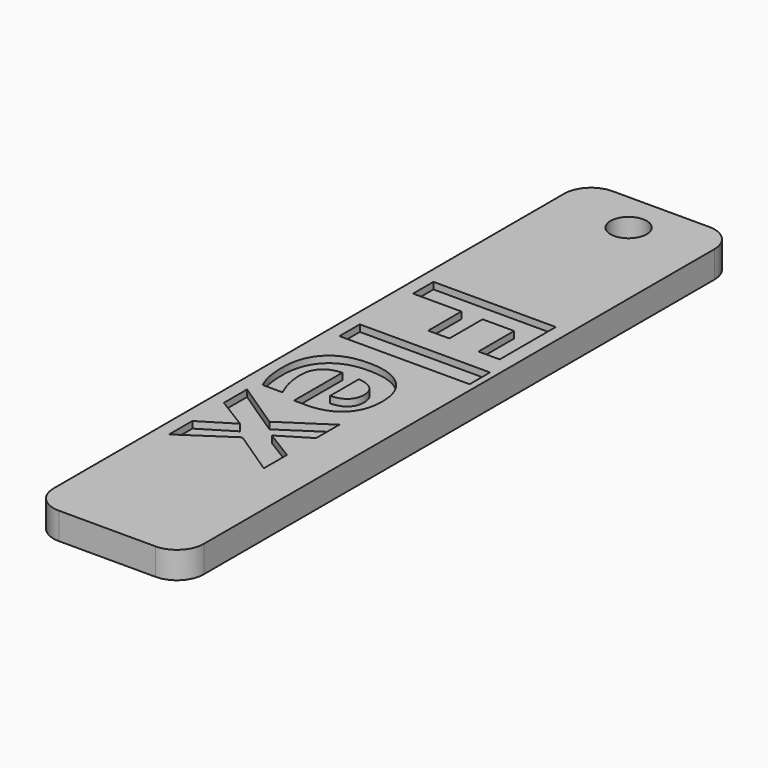
from build123d import *

# Parameters (mm, degrees)
F0_W         = 11.2
F0_H         = 51.6
F0_W_2       = 9.7091145833
F0_H_2       = 1.9026909722
F0_R         = 1.35
F0_TEXT_SIZE = 12.7777777778
F1_DEPTH     = 2
F2_DEPTH     = 0.5
F3_R         = 2


# Not quite as in the source:
# - a feature names something its author has since deleted; it is built from what else it names
# - Text() gives the source's letters only with a copy of the font that has no kerning and outlines rounded to 1/6400 em; it was checked with that copy


with BuildPart() as f1:
    # F0 (on Top) → F1 (new body)
    with BuildSketch(Plane.XY):
        with Locations((-43.6647401989, 53.6327249827)):
            Rectangle(F0_W, F0_H)
        Polygon((-48.2647401989, 46.6167961633), (-44.7029346433, 44.2509107466), (-41.2888721433, 46.4970044966), (-41.2888721433, 44.3387579688), (-43.51100756, 42.9851121355), (-41.2888721433, 41.6194871355), (-41.2888721433, 39.45924408), (-44.7029346433, 41.7312926911), (-48.2647401989, 39.3534281077), (-48.2647401989, 41.5196607466), (-45.8748964489, 42.9851121355), (-48.2647401989, 44.4565531077), align=None, mode=Mode.SUBTRACT)
        with BuildLine():
            add(Edge.make_bspline(
                [(-48.2687332544, 48.6871954688), (-48.3905214489, 49.2542093577), (-48.3905214489, 50.0727857466)],
                knots=[0, 0, 0, 1, 1, 1], degree=2))
            add(Edge.make_bspline(
                [(-48.3905214489, 50.0727857466), (-48.3905214489, 51.7558586633), (-47.4601395044, 52.7042093577)],
                knots=[0, 0, 0, 1, 1, 1], degree=2))
            add(Edge.make_bspline(
                [(-47.4601395044, 52.7042093577), (-46.52975756, 53.6525600522), (-44.8267193655, 53.6525600522)],
                knots=[0, 0, 0, 1, 1, 1], degree=2))
            add(Edge.make_bspline(
                [(-44.8267193655, 53.6525600522), (-43.0737679766, 53.6525600522), (-42.1164329072, 52.7760843577)],
                knots=[0, 0, 0, 1, 1, 1], degree=2))
            add(Edge.make_bspline(
                [(-42.1164329072, 52.7760843577), (-41.1590978377, 51.8996086633), (-41.1590978377, 50.3522996355)],
                knots=[0, 0, 0, 1, 1, 1], degree=2))
            add(Edge.make_bspline(
                [(-41.1590978377, 50.3522996355), (-41.1590978377, 48.87486908), (-42.0006342961, 48.0513013716)],
                knots=[0, 0, 0, 1, 1, 1], degree=2))
            add(Edge.make_bspline(
                [(-42.0006342961, 48.0513013716), (-42.8421707544, 47.2277336633), (-44.3275874211, 47.2277336633)],
                knots=[0, 0, 0, 1, 1, 1], degree=2))
            Line((-44.3275874211, 47.2277336633), (-45.2519797822, 47.2277336633))
            Line((-45.2519797822, 47.2277336633), (-45.2519797822, 51.7259107466))
            add(Edge.make_bspline(
                [(-45.2519797822, 51.7259107466), (-46.06257006, 51.6939663022), (-46.5177783933, 51.2447475522)],
                knots=[0, 0, 0, 1, 1, 1], degree=2))
            add(Edge.make_bspline(
                [(-46.5177783933, 51.2447475522), (-46.9729867266, 50.7955288022), (-46.9729867266, 49.9849385244)],
                knots=[0, 0, 0, 1, 1, 1], degree=2))
            add(Edge.make_bspline(
                [(-46.9729867266, 49.9849385244), (-46.9729867266, 49.3540357466), (-46.8422141572, 48.7930114411)],
                knots=[0, 0, 0, 1, 1, 1], degree=2))
            add(Edge.make_bspline(
                [(-46.8422141572, 48.7930114411), (-46.7114415877, 48.2319871355), (-46.4239415877, 47.6210496355)],
                knots=[0, 0, 0, 1, 1, 1], degree=2))
            Line((-46.4239415877, 47.6210496355), (-47.8973790877, 47.6210496355))
            add(Edge.make_bspline(
                [(-47.8973790877, 47.6210496355), (-48.14694506, 48.12018158), (-48.2687332544, 48.6871954688)],
                knots=[0, 0, 0, 1, 1, 1], degree=2))
        make_face(mode=Mode.SUBTRACT)
        Polygon((-44.6590110322, 62.0898864411), (-48.2647401989, 62.0898864411), (-48.2647401989, 63.9925774133), (-39.1426047822, 63.9925774133), (-39.1426047822, 58.7636711633), (-40.7278478377, 58.7636711633), (-40.7278478377, 62.0898864411), (-43.07975756, 62.0898864411), (-43.07975756, 58.9952683855), (-44.6590110322, 58.9952683855), align=None, mode=Mode.SUBTRACT)
        with Locations((-43.4101829072, 56.1771694272)):
            Rectangle(F0_W_2, F0_H_2, mode=Mode.SUBTRACT)
        with Locations((-43.6647401989, 76.4327249827)):
            Circle(F0_R, mode=Mode.SUBTRACT)
        with Locations(Location((-48.2647401989, 65.1405808855), (0, 0, -90))):
            Text('Flex', F0_TEXT_SIZE, font='Open Sans', font_style=FontStyle.BOLD, text_align=(TextAlign.LEFT, TextAlign.BOTTOM))
        with BuildLine():
            add(Edge.make_bspline(
                [(-42.8960770044, 49.3799906077), (-42.5127436711, 49.7353725522), (-42.5127436711, 50.3403204688)],
                knots=[0, 0, 0, 1, 1, 1], degree=2))
            add(Edge.make_bspline(
                [(-42.5127436711, 50.3403204688), (-42.5127436711, 50.9452683855), (-42.8960770044, 51.2886711633)],
                knots=[0, 0, 0, 1, 1, 1], degree=2))
            add(Edge.make_bspline(
                [(-42.8960770044, 51.2886711633), (-43.2794103377, 51.6320739411), (-43.9841846433, 51.6819871355)],
                knots=[0, 0, 0, 1, 1, 1], degree=2))
            Line((-43.9841846433, 51.6819871355), (-43.9841846433, 49.0106329688))
            add(Edge.make_bspline(
                [(-43.9841846433, 49.0106329688), (-43.2794103377, 49.0246086633), (-42.8960770044, 49.3799906077)],
                knots=[0, 0, 0, 1, 1, 1], degree=2))
        make_face()
    extrude(amount=-F1_DEPTH)

    # F0 (on Top) → F2 (cut)
    with BuildSketch(Plane.XY):
        with Locations(Location((-48.2647401989, 65.1405808855), (0, 0, -90))):
            Text('Flex', F0_TEXT_SIZE, font='Open Sans', font_style=FontStyle.BOLD, text_align=(TextAlign.LEFT, TextAlign.BOTTOM))
    extrude(amount=-F2_DEPTH, mode=Mode.SUBTRACT)

    # F3
    f3_edges = [f1.edges().sort_by_distance(p)[0] for p in [
        (-49.26474, 79.432725, -1),
        (-38.06474, 79.432725, -1),
        (-38.06474, 27.832725, -1),
        (-49.26474, 27.832725, -1),
    ]]
    fillet(f3_edges, radius=F3_R)


solid = f1.part
